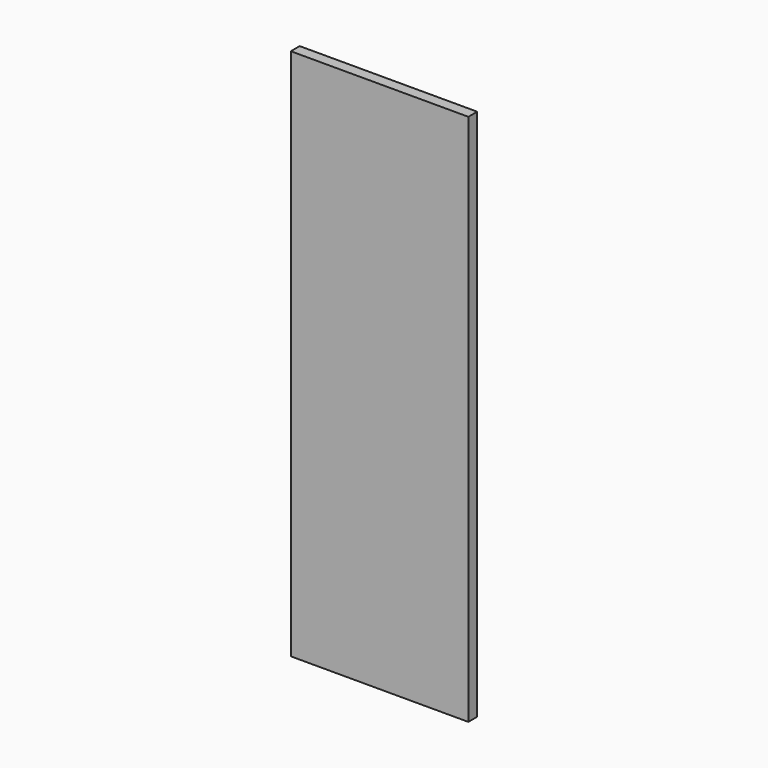
from build123d import *

# Parameters (mm, degrees)
F0_W     = 304.8
F0_H     = 914.4
F1_DEPTH = 19.05


# Not quite as in the source:
# - a length typed as a fraction of an inch, garbled in the dataset ("3 / 203.2 mm" for 3/8 in), is restored


with BuildPart() as f1:
    # F0 (on Front) → F1 (new body)
    with BuildSketch(Plane.XZ):
        with Locations((152.4, 457.2)):
            Rectangle(F0_W, F0_H)
    extrude(amount=F1_DEPTH)


solid = f1.part
